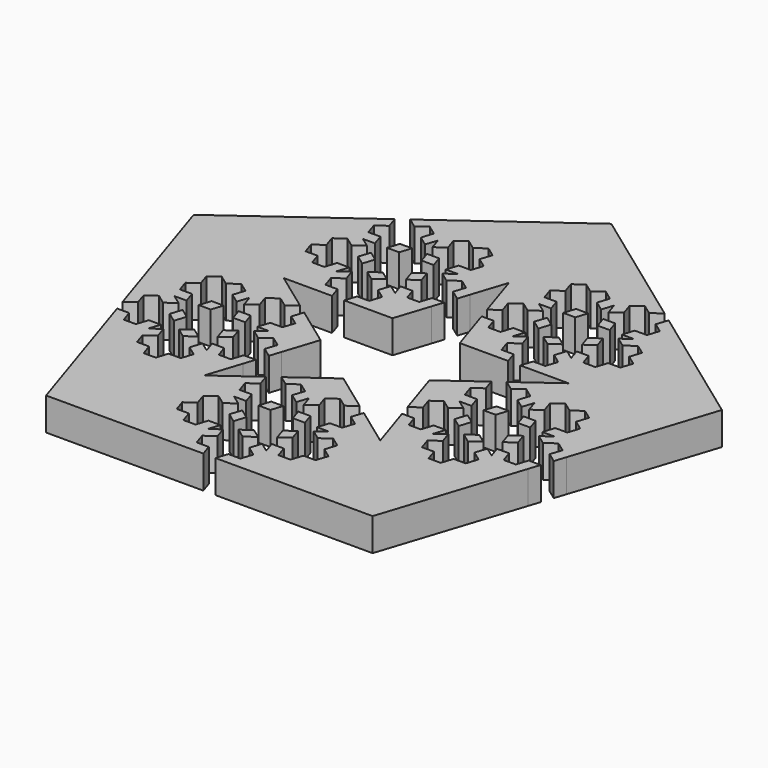
from build123d import *

# Parameters (mm, degrees)
F1_DEPTH = 25.4


with BuildPart() as f1:
    # F0 (on Top) → F1 (new body)
    with BuildSketch(Plane.XY):
        Polygon((45.6645147936, 149.7108812848), (68.4967721904, 166.299487294), (0, 216.0653053214), (-68.4967721904, 166.299487294), (-45.6645147936, 149.7108812848), (-38.053762328, 144.1813459485), (-30.4430098624, 138.6518106121), (-22.8322573968, 133.1222752757), (0, 116.5336692666), (22.8322573968, 133.1222752757), (30.4430098624, 138.6518106121), (38.053762328, 144.1813459485), align=None)
        Polygon((-45.6645147936, 149.7108812848), (-68.4967721904, 166.299487294), (-91.3290295872, 149.7108812848), (-83.7182771216, 144.1813459485), (-76.107524656, 138.6518106121), (-68.4967721904, 133.1222752757), (-60.8860197248, 138.6518106121), (-53.2752672592, 144.1813459485), align=None)
        Polygon((-8.7211462857, 89.6927409178), (0, 116.5336692666), (-22.8322573968, 133.1222752757), (-25.7393061587, 124.1752991594), (-28.6463549206, 115.2283230432), (-31.5534036825, 106.2813469269), (-23.9426512169, 100.7518115905), (-16.3318987513, 95.2222762542), align=None)
        Polygon((25.7393061587, 124.1752991594), (22.8322573968, 133.1222752757), (0, 116.5336692666), (8.7211462857, 89.6927409178), (16.3318987513, 95.2222762542), (23.9426512169, 100.7518115905), (31.5534036825, 106.2813469269), (28.6463549206, 115.2283230432), align=None)
        Polygon((83.7182771216, 144.1813459485), (91.3290295872, 149.7108812848), (68.4967721904, 166.299487294), (45.6645147936, 149.7108812848), (53.2752672592, 144.1813459485), (60.8860197248, 138.6518106121), (68.4967721904, 133.1222752757), (76.107524656, 138.6518106121), align=None)
        Polygon((-83.7182771216, 144.1813459485), (-91.3290295872, 149.7108812848), (-98.9397820528, 144.1813459485), (-91.3290295872, 138.6518106121), align=None)
        Polygon((-68.4967721904, 133.1222752757), (-76.107524656, 138.6518106121), (-79.0145734179, 129.7048344958), (-71.4038209523, 124.1752991594), align=None)
        Polygon((-57.9789709629, 129.7048344958), (-60.8860197248, 138.6518106121), (-68.4967721904, 133.1222752757), (-65.5897234285, 124.1752991594), align=None)
        Polygon((-38.053762328, 144.1813459485), (-45.6645147936, 149.7108812848), (-53.2752672592, 144.1813459485), (-45.6645147936, 138.6518106121), align=None)
        Polygon((-22.8322573968, 133.1222752757), (-30.4430098624, 138.6518106121), (-33.3500586243, 129.7048344958), (-25.7393061587, 124.1752991594), align=None)
        Polygon((-31.5534036825, 106.2813469269), (-28.6463549206, 115.2283230432), (-38.053762328, 115.2283230432), (-40.9608110899, 106.2813469269), align=None)
        Polygon((-31.5534036825, 95.2222762542), (-23.9426512169, 100.7518115905), (-31.5534036825, 106.2813469269), (-39.1641561481, 100.7518115905), align=None)
        Polygon((-11.6281950476, 80.7457648015), (-8.7211462857, 89.6927409178), (-16.3318987513, 95.2222762542), (-19.2389475132, 86.2753001379), align=None)
        Polygon((16.3318987513, 95.2222762542), (8.7211462857, 89.6927409178), (11.6281950476, 80.7457648015), (19.2389475132, 86.2753001379), align=None)
        Polygon((39.1641561481, 100.7518115905), (31.5534036825, 106.2813469269), (23.9426512169, 100.7518115905), (31.5534036825, 95.2222762542), align=None)
        Polygon((38.053762328, 115.2283230432), (28.6463549206, 115.2283230432), (31.5534036825, 106.2813469269), (40.9608110899, 106.2813469269), align=None)
        Polygon((33.3500586243, 129.7048344958), (30.4430098624, 138.6518106121), (22.8322573968, 133.1222752757), (25.7393061587, 124.1752991594), align=None)
        Polygon((53.2752672592, 144.1813459485), (45.6645147936, 149.7108812848), (38.053762328, 144.1813459485), (45.6645147936, 138.6518106121), align=None)
        Polygon((65.5897234285, 124.1752991594), (68.4967721904, 133.1222752757), (60.8860197248, 138.6518106121), (57.9789709629, 129.7048344958), align=None)
        Polygon((79.0145734179, 129.7048344958), (76.107524656, 138.6518106121), (68.4967721904, 133.1222752757), (71.4038209523, 124.1752991594), align=None)
        Polygon((91.3290295872, 138.6518106121), (98.9397820528, 144.1813459485), (91.3290295872, 149.7108812848), (83.7182771216, 144.1813459485), align=None)
    extrude(amount=F1_DEPTH)


with BuildPart() as f1b:
    # F0 (on Top) → F1, piece 2 (new body)
    with BuildSketch(Plane.XY):
        Polygon((156.4946203174, 2.8336722019), (179.3268777142, -13.7549338072), (205.4903165712, 66.7678512391), (136.9935443808, 116.5336692666), (128.2723980951, 89.6927409178), (125.3653493332, 80.7457648015), (122.4583005713, 71.7987886853), (119.5512518094, 62.851812569), (110.8301055237, 36.0108842202), (133.6623629205, 19.4222782111), (141.2731153862, 13.8927428747), (148.8838678518, 8.3632075383), align=None)
        Polygon((128.2723980951, 89.6927409178), (136.9935443808, 116.5336692666), (114.161286984, 133.1222752757), (111.2542382221, 124.1752991594), (108.3471894602, 115.2283230432), (105.4401406983, 106.2813469269), (113.0508931639, 100.7518115905), (120.6616456295, 95.2222762542), align=None)
        Polygon((82.6078833015, 36.0108842202), (110.8301055237, 36.0108842202), (119.5512518094, 62.851812569), (110.143844402, 62.851812569), (100.7364369946, 62.851812569), (91.3290295872, 62.851812569), (88.4219808253, 53.9048364528), (85.5149320634, 44.9578603365), align=None)
        Polygon((126.0516104549, 13.8927428747), (133.6623629205, 19.4222782111), (110.8301055237, 36.0108842202), (87.9978481269, 19.4222782111), (95.6086005925, 13.8927428747), (103.2193530581, 8.3632075383), (110.8301055237, 2.833672202), (118.4408579893, 8.3632075383), align=None)
        Polygon((162.9949789629, -35.0663268196), (170.6057314285, -40.595862156), (179.3268777142, -13.7549338072), (156.4946203174, 2.8336722019), (153.5875715555, -6.1133039143), (150.6805227936, -15.0602800306), (147.7734740317, -24.0072561468), (155.3842264973, -29.5367914832), align=None)
        Polygon((111.2542382221, 124.1752991594), (114.161286984, 133.1222752757), (106.5505345184, 138.6518106121), (103.6434857565, 129.7048344958), align=None)
        Polygon((105.4401406983, 106.2813469269), (108.3471894602, 115.2283230432), (98.9397820528, 115.2283230432), (96.0327332909, 106.2813469269), align=None)
        Polygon((105.4401406983, 95.2222762542), (113.0508931639, 100.7518115905), (105.4401406983, 106.2813469269), (97.8293882327, 100.7518115905), align=None)
        Polygon((125.3653493332, 80.7457648015), (128.2723980951, 89.6927409178), (120.6616456295, 95.2222762542), (117.7545968676, 86.2753001379), align=None)
        Polygon((119.5512518094, 62.851812569), (122.4583005713, 71.7987886853), (113.0508931639, 71.7987886853), (110.143844402, 62.851812569), align=None)
        Polygon((91.3290295872, 62.851812569), (100.7364369946, 62.851812569), (97.8293882327, 71.7987886853), (88.4219808253, 71.7987886853), align=None)
        Polygon((80.8112283597, 59.4343717891), (88.4219808253, 53.9048364528), (91.3290295872, 62.851812569), (83.7182771216, 68.3813479054), align=None)
        Polygon((73.2004758941, 36.0108842202), (82.6078833015, 36.0108842202), (85.5149320634, 44.9578603365), (76.107524656, 44.9578603365), align=None)
        Polygon((95.6086005925, 13.8927428747), (87.9978481269, 19.4222782111), (80.3870956613, 13.8927428747), (87.9978481269, 8.3632075383), align=None)
        Polygon((107.9230567618, -6.1133039143), (110.8301055237, 2.833672202), (103.2193530581, 8.3632075383), (100.3123042962, -0.5837685779), align=None)
        Polygon((121.3479067512, -0.5837685779), (118.4408579893, 8.3632075383), (110.8301055237, 2.833672202), (113.7371542856, -6.1133039143), align=None)
        Polygon((133.6623629205, 8.3632075383), (141.2731153862, 13.8927428747), (133.6623629205, 19.4222782111), (126.0516104549, 13.8927428747), align=None)
        Polygon((153.5875715555, -6.1133039143), (156.4946203174, 2.833672202), (148.8838678518, 8.3632075383), (145.9768190899, -0.5837685779), align=None)
        Polygon((138.3660666243, -24.0072561468), (147.7734740317, -24.0072561468), (150.6805227936, -15.0602800306), (141.2731153862, -15.0602800306), align=None)
        Polygon((147.7734740317, -35.0663268196), (155.3842264973, -29.5367914832), (147.7734740317, -24.0072561468), (140.1627215661, -29.5367914832), align=None)
        Polygon((160.087930201, -44.0133029358), (167.6986826666, -49.5428382722), (170.6057314285, -40.595862156), (162.9949789629, -35.0663268196), align=None)
    extrude(amount=F1_DEPTH)


with BuildPart() as f1c:
    # F0 (on Top) → F1, piece 3 (new body)
    with BuildSketch(Plane.XY):
        Polygon((42.3333333333, -174.8005038998), (127, -174.8005038998), (153.1634388571, -94.2777188535), (124.9412166349, -94.2777188535), (115.5338092274, -94.2777188535), (106.12640182, -94.2777188535), (96.7189944126, -94.2777188535), (68.4967721904, -94.2777188535), (59.7756259047, -121.1186472023), (56.8685771428, -130.0656233185), (53.9615283809, -139.0125994348), (51.054479619, -147.9595755511), align=None)
        Polygon((124.9412166349, -94.2777188535), (153.1634388571, -94.2777188535), (161.8845851428, -67.4367905047), (152.4771777354, -67.4367905047), (143.069770328, -67.4367905047), (133.6623629205, -67.4367905047), (130.7553141587, -76.383766621), (127.8482653968, -85.3307427373), align=None)
        Polygon((68.4967721904, -94.2777188535), (96.7189944126, -94.2777188535), (93.8119456507, -85.3307427373), (90.9048968888, -76.383766621), (87.9978481269, -67.4367905047), (78.5904407195, -67.4367905047), (69.1830333121, -67.4367905047), (59.7756259047, -67.4367905047), align=None)
        Polygon((52.1648734391, -115.5891118659), (59.7756259047, -121.1186472023), (68.4967721904, -94.2777188535), (45.6645147936, -77.6891128444), (42.7574660317, -86.6360889606), (39.8504172698, -95.5830650769), (36.9433685079, -104.5300411931), (44.5541209735, -110.0595765295), align=None)
        Polygon((14.1111111111, -174.8005038998), (42.3333333333, -174.8005038998), (51.054479619, -147.9595755511), (41.6470722116, -147.9595755511), (32.2396648042, -147.9595755511), (22.8322573968, -147.9595755511), (19.9252086349, -156.9065516673), (17.018159873, -165.8535277836), align=None)
        Polygon((152.4771777354, -67.4367905047), (161.8845851428, -67.4367905047), (164.7916339047, -58.4898143885), (155.3842264973, -58.4898143885), align=None)
        Polygon((133.6623629205, -67.4367905047), (143.069770328, -67.4367905047), (140.1627215661, -58.4898143885), (130.7553141587, -58.4898143885), align=None)
        Polygon((123.1445616931, -70.8542312846), (130.7553141587, -76.383766621), (133.6623629205, -67.4367905047), (126.0516104549, -61.9072551684), align=None)
        Polygon((115.5338092274, -94.2777188535), (124.9412166349, -94.2777188535), (127.8482653968, -85.3307427373), (118.4408579893, -85.3307427373), align=None)
        Polygon((96.7189944126, -94.2777188535), (106.12640182, -94.2777188535), (103.2193530581, -85.3307427373), (93.8119456507, -85.3307427373), align=None)
        Polygon((87.9978481269, -67.4367905047), (90.9048968888, -76.383766621), (98.5156493544, -70.8542312846), (95.6086005925, -61.9072551684), align=None)
        Polygon((78.5904407195, -67.4367905047), (87.9978481269, -67.4367905047), (90.9048968888, -58.4898143885), (81.4974894814, -58.4898143885), align=None)
        Polygon((56.8685771428, -58.4898143885), (59.7756259047, -67.4367905047), (69.1830333121, -67.4367905047), (66.2759845502, -58.4898143885), align=None)
        Polygon((42.7574660317, -86.6360889606), (45.6645147936, -77.6891128444), (38.053762328, -72.159577508), (35.1467135661, -81.1065536242), align=None)
        Polygon((27.5359611005, -104.5300411931), (36.9433685079, -104.5300411931), (39.8504172698, -95.5830650769), (30.4430098624, -95.5830650769), align=None)
        Polygon((36.9433685079, -115.5891118659), (44.5541209735, -110.0595765295), (36.9433685079, -104.5300411931), (29.3326160423, -110.0595765295), align=None)
        Polygon((49.2578246772, -124.5360879822), (56.8685771428, -130.0656233185), (59.7756259047, -121.1186472023), (52.1648734391, -115.5891118659), align=None)
        Polygon((41.6470722116, -147.9595755511), (51.054479619, -147.9595755511), (53.9615283809, -139.0125994348), (44.5541209735, -139.0125994348), align=None)
        Polygon((22.8322573968, -147.9595755511), (32.2396648042, -147.9595755511), (29.3326160423, -139.0125994348), (19.9252086349, -139.0125994348), align=None)
        Polygon((12.3144561693, -151.3770163309), (19.9252086349, -156.9065516673), (22.8322573968, -147.9595755511), (15.2215049312, -142.4300402147), align=None)
        Polygon((4.7037037037, -174.8005038998), (14.1111111111, -174.8005038998), (17.018159873, -165.8535277836), (7.6107524656, -165.8535277836), align=None)
    extrude(amount=F1_DEPTH)


with BuildPart() as f1d:
    # F0 (on Top) → F1, piece 4 (new body)
    with BuildSketch(Plane.XY):
        Polygon((-127, -174.8005038998), (-42.3333333333, -174.8005038998), (-51.054479619, -147.9595755511), (-53.9615283809, -139.0125994348), (-56.8685771428, -130.0656233185), (-59.7756259047, -121.1186472023), (-68.4967721904, -94.2777188535), (-96.7189944126, -94.2777188535), (-106.12640182, -94.2777188535), (-115.5338092274, -94.2777188535), (-124.9412166349, -94.2777188535), (-153.1634388571, -94.2777188535), align=None)
        Polygon((-42.3333333333, -174.8005038998), (-14.1111111111, -174.8005038998), (-17.018159873, -165.8535277836), (-19.9252086349, -156.9065516673), (-22.8322573968, -147.9595755511), (-32.2396648042, -147.9595755511), (-41.6470722116, -147.9595755511), (-51.054479619, -147.9595755511), align=None)
        Polygon((-68.4967721904, -94.2777188535), (-59.7756259047, -121.1186472023), (-52.1648734391, -115.5891118659), (-44.5541209735, -110.0595765295), (-36.9433685079, -104.5300411931), (-39.8504172698, -95.5830650769), (-42.7574660317, -86.6360889606), (-45.6645147936, -77.6891128444), align=None)
        Polygon((-96.7189944126, -94.2777188535), (-68.4967721904, -94.2777188535), (-59.7756259047, -67.4367905047), (-69.1830333121, -67.4367905047), (-78.5904407195, -67.4367905047), (-87.9978481269, -67.4367905047), (-90.9048968888, -76.383766621), (-93.8119456507, -85.3307427373), align=None)
        Polygon((-161.8845851428, -67.4367905047), (-153.1634388571, -94.2777188535), (-124.9412166349, -94.2777188535), (-127.8482653968, -85.3307427373), (-130.7553141587, -76.383766621), (-133.6623629205, -67.4367905047), (-143.069770328, -67.4367905047), (-152.4771777354, -67.4367905047), align=None)
        Polygon((-14.1111111111, -174.8005038998), (-4.7037037037, -174.8005038998), (-7.6107524656, -165.8535277836), (-17.018159873, -165.8535277836), align=None)
        Polygon((-22.8322573968, -147.9595755511), (-19.9252086349, -156.9065516673), (-12.3144561693, -151.3770163309), (-15.2215049312, -142.4300402147), align=None)
        Polygon((-32.2396648042, -147.9595755511), (-22.8322573968, -147.9595755511), (-19.9252086349, -139.0125994348), (-29.3326160423, -139.0125994348), align=None)
        Polygon((-53.9615283809, -139.0125994348), (-51.054479619, -147.9595755511), (-41.6470722116, -147.9595755511), (-44.5541209735, -139.0125994348), align=None)
        Polygon((-59.7756259047, -121.1186472023), (-56.8685771428, -130.0656233185), (-49.2578246772, -124.5360879822), (-52.1648734391, -115.5891118659), align=None)
        Polygon((-36.9433685079, -104.5300411931), (-44.5541209735, -110.0595765295), (-36.9433685079, -115.5891118659), (-29.3326160423, -110.0595765295), align=None)
        Polygon((-39.8504172698, -95.5830650769), (-36.9433685079, -104.5300411931), (-27.5359611005, -104.5300411931), (-30.4430098624, -95.5830650769), align=None)
        Polygon((-38.053762328, -72.159577508), (-45.6645147936, -77.6891128444), (-42.7574660317, -86.6360889606), (-35.1467135661, -81.1065536243), align=None)
        Polygon((-140.1627215661, -58.4898143885), (-143.069770328, -67.4367905047), (-133.6623629205, -67.4367905047), (-130.7553141587, -58.4898143885), align=None)
        Polygon((-164.7916339047, -58.4898143885), (-161.8845851428, -67.4367905047), (-152.4771777354, -67.4367905047), (-155.3842264973, -58.4898143885), align=None)
        Polygon((-87.9978481269, -67.4367905047), (-78.5904407195, -67.4367905047), (-81.4974894814, -58.4898143885), (-90.9048968888, -58.4898143885), align=None)
        Polygon((-69.1830333121, -67.4367905047), (-59.7756259047, -67.4367905047), (-56.8685771428, -58.4898143885), (-66.2759845502, -58.4898143885), align=None)
        Polygon((-103.2193530581, -85.3307427373), (-106.12640182, -94.2777188535), (-96.7189944126, -94.2777188535), (-93.8119456507, -85.3307427373), align=None)
        Polygon((-127.8482653968, -85.3307427373), (-124.9412166349, -94.2777188535), (-115.5338092274, -94.2777188535), (-118.4408579893, -85.3307427373), align=None)
        Polygon((-133.6623629205, -67.4367905047), (-130.7553141587, -76.383766621), (-123.1445616931, -70.8542312846), (-126.0516104549, -61.9072551684), align=None)
        Polygon((-98.5156493544, -70.8542312846), (-90.9048968888, -76.383766621), (-87.9978481269, -67.4367905047), (-95.6086005925, -61.9072551684), align=None)
    extrude(amount=F1_DEPTH)


with BuildPart() as f1e:
    # F0 (on Top) → F1, piece 5 (new body)
    with BuildSketch(Plane.XY):
        Polygon((-205.4903165712, 66.7678512391), (-179.3268777142, -13.7549338072), (-156.4946203174, 2.833672202), (-148.8838678518, 8.3632075383), (-141.2731153862, 13.8927428747), (-133.6623629205, 19.4222782111), (-110.8301055237, 36.0108842202), (-119.5512518094, 62.851812569), (-122.4583005713, 71.7987886853), (-125.3653493332, 80.7457648015), (-128.2723980951, 89.6927409178), (-136.9935443808, 116.5336692666), align=None)
        Polygon((-114.161286984, 133.1222752757), (-136.9935443808, 116.5336692666), (-128.2723980951, 89.6927409178), (-120.6616456295, 95.2222762542), (-113.0508931639, 100.7518115905), (-105.4401406983, 106.2813469269), (-108.3471894602, 115.2283230432), (-111.2542382221, 124.1752991594), align=None)
        Polygon((-179.3268777142, -13.7549338072), (-170.6057314285, -40.595862156), (-162.9949789629, -35.0663268196), (-155.3842264973, -29.5367914832), (-147.7734740317, -24.0072561468), (-150.6805227936, -15.0602800306), (-153.5875715555, -6.1133039143), (-156.4946203174, 2.833672202), align=None)
        Polygon((-110.8301055237, 36.0108842202), (-133.6623629205, 19.4222782111), (-126.0516104549, 13.8927428747), (-118.4408579893, 8.3632075383), (-110.8301055237, 2.833672202), (-103.2193530581, 8.3632075383), (-95.6086005925, 13.8927428747), (-87.9978481269, 19.4222782111), align=None)
        Polygon((-119.5512518094, 62.851812569), (-110.8301055237, 36.0108842202), (-82.6078833015, 36.0108842202), (-85.5149320634, 44.9578603365), (-88.4219808253, 53.9048364528), (-91.3290295872, 62.851812569), (-100.7364369946, 62.851812569), (-110.143844402, 62.851812569), align=None)
        Polygon((-106.5505345184, 138.6518106121), (-114.161286984, 133.1222752757), (-111.2542382221, 124.1752991594), (-103.6434857565, 129.7048344958), align=None)
        Polygon((-98.9397820528, 115.2283230432), (-108.3471894602, 115.2283230432), (-105.4401406983, 106.2813469269), (-96.0327332909, 106.2813469269), align=None)
        Polygon((-105.4401406983, 106.2813469269), (-113.0508931639, 100.7518115905), (-105.4401406983, 95.2222762542), (-97.8293882327, 100.7518115905), align=None)
        Polygon((-120.6616456295, 95.2222762542), (-128.2723980951, 89.6927409178), (-125.3653493332, 80.7457648015), (-117.7545968676, 86.2753001379), align=None)
        Polygon((-113.0508931639, 71.7987886853), (-122.4583005713, 71.7987886853), (-119.5512518094, 62.851812569), (-110.143844402, 62.851812569), align=None)
        Polygon((-97.8293882327, 71.7987886853), (-100.7364369946, 62.851812569), (-91.3290295872, 62.851812569), (-88.4219808253, 71.7987886853), align=None)
        Polygon((-91.3290295872, 62.851812569), (-88.4219808253, 53.9048364528), (-80.8112283597, 59.4343717891), (-83.7182771216, 68.3813479054), align=None)
        Polygon((-85.5149320634, 44.9578603365), (-82.6078833015, 36.0108842202), (-73.2004758941, 36.0108842202), (-76.107524656, 44.9578603365), align=None)
        Polygon((-170.6057314285, -40.595862156), (-167.6986826666, -49.5428382722), (-160.087930201, -44.0133029358), (-162.9949789629, -35.0663268196), align=None)
        Polygon((-147.7734740317, -24.0072561468), (-155.3842264973, -29.5367914832), (-147.7734740317, -35.0663268196), (-140.1627215661, -29.5367914832), align=None)
        Polygon((-150.6805227936, -15.0602800306), (-147.7734740317, -24.0072561468), (-138.3660666243, -24.0072561468), (-141.2731153862, -15.0602800306), align=None)
        Polygon((-148.8838678518, 8.3632075383), (-156.4946203174, 2.833672202), (-153.5875715555, -6.1133039143), (-145.9768190899, -0.5837685779), align=None)
        Polygon((-133.6623629205, 19.4222782111), (-141.2731153862, 13.8927428747), (-133.6623629205, 8.3632075383), (-126.0516104549, 13.8927428747), align=None)
        Polygon((-110.8301055237, 2.833672202), (-118.4408579893, 8.3632075383), (-121.3479067512, -0.5837685779), (-113.7371542856, -6.1133039143), align=None)
        Polygon((-103.2193530581, 8.3632075383), (-110.8301055237, 2.833672202), (-107.9230567618, -6.1133039143), (-100.3123042962, -0.5837685779), align=None)
        Polygon((-80.3870956613, 13.8927428747), (-87.9978481269, 19.4222782111), (-95.6086005925, 13.8927428747), (-87.9978481269, 8.3632075383), align=None)
    extrude(amount=F1_DEPTH)


with BuildPart() as f1f:
    # F0 (on Top) → F1, piece 6 (new body)
    with BuildSketch(Plane.XY):
        Polygon((-51.4786123174, 44.9578603365), (-54.3856610793, 36.0108842202), (-26.1634388571, 36.0108842202), (-17.4422925714, 62.851812569), (-26.8496999788, 62.851812569), (-36.2571073862, 62.851812569), (-45.6645147936, 62.851812569), (-48.5715635555, 53.9048364528), align=None)
        Polygon((-17.4422925714, 62.851812569), (-14.5352438095, 71.7987886853), (-23.9426512169, 71.7987886853), (-26.8496999788, 62.851812569), align=None)
        Polygon((-45.6645147936, 62.851812569), (-36.2571073862, 62.851812569), (-39.1641561481, 71.7987886853), (-48.5715635555, 71.7987886853), align=None)
        Polygon((-56.1823160211, 59.4343717891), (-48.5715635555, 53.9048364528), (-45.6645147936, 62.851812569), (-53.2752672592, 68.3813479054), align=None)
        Polygon((-60.8860197248, 44.9578603365), (-63.7930684867, 36.0108842202), (-54.3856610793, 36.0108842202), (-51.4786123174, 44.9578603365), align=None)
    extrude(amount=F1_DEPTH)


with BuildPart() as f1g:
    # F0 (on Top) → F1, piece 7 (new body)
    with BuildSketch(Plane.XY):
        Polygon((26.1634388571, 36.0108842202), (54.3856610793, 36.0108842202), (51.4786123174, 44.9578603365), (48.5715635555, 53.9048364528), (45.6645147936, 62.851812569), (36.2571073862, 62.851812569), (26.8496999788, 62.851812569), (17.4422925714, 62.851812569), align=None)
        Polygon((54.3856610793, 36.0108842202), (63.7930684867, 36.0108842202), (60.8860197248, 44.9578603365), (51.4786123174, 44.9578603365), align=None)
        Polygon((45.6645147936, 62.851812569), (48.5715635555, 53.9048364528), (56.1823160211, 59.4343717891), (53.2752672592, 68.3813479054), align=None)
        Polygon((36.2571073862, 62.851812569), (45.6645147936, 62.851812569), (48.5715635555, 71.7987886853), (39.1641561481, 71.7987886853), align=None)
        Polygon((14.5352438095, 71.7987886853), (17.4422925714, 62.851812569), (26.8496999788, 62.851812569), (23.9426512169, 71.7987886853), align=None)
    extrude(amount=F1_DEPTH)


with BuildPart() as f1h:
    # F0 (on Top) → F1, piece 8 (new body)
    with BuildSketch(Plane.XY):
        Polygon((42.3333333333, -13.7549338072), (51.054479619, -40.595862156), (58.6652320846, -35.0663268196), (66.2759845502, -29.5367914832), (73.8867370158, -24.0072561468), (70.9796882539, -15.0602800306), (68.072639492, -6.1133039143), (65.1655907301, 2.833672202), align=None)
        Polygon((51.054479619, -40.595862156), (53.9615283809, -49.5428382722), (61.5722808465, -44.0133029358), (58.6652320846, -35.0663268196), align=None)
        Polygon((73.8867370158, -24.0072561468), (66.2759845502, -29.5367914832), (73.8867370158, -35.0663268196), (81.4974894814, -29.5367914832), align=None)
        Polygon((70.9796882539, -15.0602800306), (73.8867370158, -24.0072561468), (83.2941444232, -24.0072561468), (80.3870956613, -15.0602800306), align=None)
        Polygon((72.7763431957, 8.3632075383), (65.1655907301, 2.833672202), (68.072639492, -6.1133039143), (75.6833919576, -0.5837685779), align=None)
    extrude(amount=F1_DEPTH)


with BuildPart() as f1i:
    # F0 (on Top) → F1, piece 9 (new body)
    with BuildSketch(Plane.XY):
        Polygon((15.2215049312, -66.6300421716), (22.8322573968, -61.1005068352), (0, -44.5119008261), (-22.8322573968, -61.1005068352), (-15.2215049312, -66.6300421716), (-7.6107524656, -72.159577508), (0, -77.6891128444), (7.6107524656, -72.159577508), align=None)
        Polygon((22.8322573968, -72.159577508), (30.4430098624, -66.6300421716), (22.8322573968, -61.1005068352), (15.2215049312, -66.6300421716), align=None)
        Polygon((-15.2215049312, -66.6300421716), (-22.8322573968, -61.1005068352), (-30.4430098624, -66.6300421716), (-22.8322573968, -72.159577508), align=None)
        Polygon((-2.9070487619, -86.6360889606), (0, -77.6891128444), (-7.6107524656, -72.159577508), (-10.5178012275, -81.1065536242), align=None)
        Polygon((10.5178012275, -81.1065536242), (7.6107524656, -72.159577508), (0, -77.6891128444), (2.9070487619, -86.6360889606), align=None)
    extrude(amount=F1_DEPTH)


with BuildPart() as f1j:
    # F0 (on Top) → F1, piece 10 (new body)
    with BuildSketch(Plane.XY):
        Polygon((-58.6652320846, -35.0663268196), (-51.054479619, -40.595862156), (-42.3333333333, -13.7549338072), (-65.1655907301, 2.833672202), (-68.072639492, -6.1133039143), (-70.9796882539, -15.0602800306), (-73.8867370158, -24.0072561468), (-66.2759845502, -29.5367914832), align=None)
        Polygon((-68.072639492, -6.1133039143), (-65.1655907301, 2.833672202), (-72.7763431957, 8.3632075383), (-75.6833919576, -0.5837685779), align=None)
        Polygon((-83.2941444232, -24.0072561468), (-73.8867370158, -24.0072561468), (-70.9796882539, -15.0602800306), (-80.3870956613, -15.0602800306), align=None)
        Polygon((-73.8867370158, -35.0663268196), (-66.2759845502, -29.5367914832), (-73.8867370158, -24.0072561468), (-81.4974894814, -29.5367914832), align=None)
        Polygon((-61.5722808465, -44.0133029358), (-53.9615283809, -49.5428382722), (-51.054479619, -40.595862156), (-58.6652320846, -35.0663268196), align=None)
    extrude(amount=F1_DEPTH)


with BuildPart() as f1k:
    # F0 (on Top) → F1, piece 11 (new body)
    with BuildSketch(Plane.XY):
        Polygon((59.7756259047, 106.2813469269), (62.6826746666, 115.2283230432), (53.2752672592, 115.2283230432), (50.3682184973, 106.2813469269), align=None)
    extrude(amount=F1_DEPTH)


with BuildPart() as f1l:
    # F0 (on Top) → F1, piece 12 (new body)
    with BuildSketch(Plane.XY):
        Polygon((86.6253258835, 106.2813469269), (83.7182771216, 115.2283230432), (74.3108697142, 115.2283230432), (77.2179184761, 106.2813469269), align=None)
    extrude(amount=F1_DEPTH)


with BuildPart() as f1m:
    # F0 (on Top) → F1, piece 13 (new body)
    with BuildSketch(Plane.XY):
        Polygon((93.125684529, 86.2753001379), (90.2186357671, 95.2222762542), (82.6078833015, 89.6927409178), (85.5149320634, 80.7457648015), align=None)
    extrude(amount=F1_DEPTH)


with BuildPart() as f1n:
    # F0 (on Top) → F1, piece 14 (new body)
    with BuildSketch(Plane.XY):
        Polygon((68.4967721904, 68.3813479054), (76.107524656, 73.9108832418), (68.4967721904, 79.4404185782), (60.8860197248, 73.9108832418), align=None)
    extrude(amount=F1_DEPTH)


with BuildPart() as f1o:
    # F0 (on Top) → F1, piece 15 (new body)
    with BuildSketch(Plane.XY):
        Polygon((43.8678598518, 86.2753001379), (51.4786123174, 80.7457648015), (54.3856610793, 89.6927409178), (46.7749086137, 95.2222762542), align=None)
    extrude(amount=F1_DEPTH)


with BuildPart() as f1p:
    # F0 (on Top) → F1, piece 16 (new body)
    with BuildSketch(Plane.XY):
        Polygon((-43.8678598518, 86.2753001379), (-46.7749086137, 95.2222762542), (-54.3856610793, 89.6927409178), (-51.4786123174, 80.7457648015), align=None)
    extrude(amount=F1_DEPTH)


with BuildPart() as f1q:
    # F0 (on Top) → F1, piece 17 (new body)
    with BuildSketch(Plane.XY):
        Polygon((-53.2752672592, 115.2283230432), (-62.6826746666, 115.2283230432), (-59.7756259047, 106.2813469269), (-50.3682184973, 106.2813469269), align=None)
    extrude(amount=F1_DEPTH)


with BuildPart() as f1r:
    # F0 (on Top) → F1, piece 18 (new body)
    with BuildSketch(Plane.XY):
        Polygon((-74.3108697142, 115.2283230432), (-83.7182771216, 115.2283230432), (-86.6253258835, 106.2813469269), (-77.2179184761, 106.2813469269), align=None)
    extrude(amount=F1_DEPTH)


with BuildPart() as f1s:
    # F0 (on Top) → F1, piece 19 (new body)
    with BuildSketch(Plane.XY):
        Polygon((-82.6078833015, 89.6927409178), (-90.2186357671, 95.2222762542), (-93.125684529, 86.2753001379), (-85.5149320634, 80.7457648015), align=None)
    extrude(amount=F1_DEPTH)


with BuildPart() as f1t:
    # F0 (on Top) → F1, piece 20 (new body)
    with BuildSketch(Plane.XY):
        Polygon((-68.4967721904, 79.4404185782), (-76.107524656, 73.9108832418), (-68.4967721904, 68.3813479054), (-60.8860197248, 73.9108832418), align=None)
    extrude(amount=F1_DEPTH)


with BuildPart() as f1u:
    # F0 (on Top) → F1, piece 21 (new body)
    with BuildSketch(Plane.XY):
        Polygon((95.6086005925, -15.0602800306), (92.7015518306, -24.0072561468), (102.1089592381, -24.0072561468), (105.016008, -15.0602800306), align=None)
    extrude(amount=F1_DEPTH)


with BuildPart() as f1v:
    # F0 (on Top) → F1, piece 22 (new body)
    with BuildSketch(Plane.XY):
        Polygon((119.5512518094, -24.0072561468), (128.9586592168, -24.0072561468), (126.0516104549, -15.0602800306), (116.6442030475, -15.0602800306), align=None)
    extrude(amount=F1_DEPTH)


with BuildPart() as f1w:
    # F0 (on Top) → F1, piece 23 (new body)
    with BuildSketch(Plane.XY):
        Polygon((127.8482653968, -49.5428382722), (135.4590178624, -44.0133029358), (132.5519691005, -35.0663268196), (124.9412166349, -40.595862156), align=None)
    extrude(amount=F1_DEPTH)


with BuildPart() as f1x:
    # F0 (on Top) → F1, piece 24 (new body)
    with BuildSketch(Plane.XY):
        Polygon((110.8301055237, -61.9072551684), (118.4408579893, -56.377719832), (110.8301055237, -50.8481844956), (103.2193530581, -56.377719832), align=None)
    extrude(amount=F1_DEPTH)


with BuildPart() as f1y:
    # F0 (on Top) → F1, piece 25 (new body)
    with BuildSketch(Plane.XY):
        Polygon((86.2011931851, -44.0133029358), (93.8119456507, -49.5428382722), (96.7189944126, -40.595862156), (89.108241947, -35.0663268196), align=None)
    extrude(amount=F1_DEPTH)


with BuildPart() as f1z:
    # F0 (on Top) → F1, piece 26 (new body)
    with BuildSketch(Plane.XY):
        Polygon((14.1111111111, -121.1186472023), (17.018159873, -130.0656233185), (24.6289123386, -124.5360879822), (21.7218635767, -115.5891118659), align=None)
    extrude(amount=F1_DEPTH)


with BuildPart() as f1ba:
    # F0 (on Top) → F1, piece 27 (new body)
    with BuildSketch(Plane.XY):
        Polygon((0, -142.4300402147), (7.6107524656, -136.9005048783), (0, -131.3709695419), (-7.6107524656, -136.9005048783), align=None)
    extrude(amount=F1_DEPTH)


with BuildPart() as f1bb:
    # F0 (on Top) → F1, piece 28 (new body)
    with BuildSketch(Plane.XY):
        Polygon((-24.6289123386, -124.5360879822), (-17.018159873, -130.0656233185), (-14.1111111111, -121.1186472023), (-21.7218635767, -115.5891118659), align=None)
    extrude(amount=F1_DEPTH)


with BuildPart() as f1bc:
    # F0 (on Top) → F1, piece 29 (new body)
    with BuildSketch(Plane.XY):
        Polygon((-15.2215049312, -95.5830650769), (-18.1285536931, -104.5300411931), (-8.7211462857, -104.5300411931), (-5.8140975238, -95.5830650769), align=None)
    extrude(amount=F1_DEPTH)


with BuildPart() as f1bd:
    # F0 (on Top) → F1, piece 30 (new body)
    with BuildSketch(Plane.XY):
        Polygon((8.7211462857, -104.5300411931), (18.1285536931, -104.5300411931), (15.2215049312, -95.5830650769), (5.8140975238, -95.5830650769), align=None)
    extrude(amount=F1_DEPTH)


with BuildPart() as f1be:
    # F0 (on Top) → F1, piece 31 (new body)
    with BuildSketch(Plane.XY):
        Polygon((-132.5519691005, -35.0663268196), (-135.4590178624, -44.0133029358), (-127.8482653968, -49.5428382722), (-124.9412166349, -40.595862156), align=None)
    extrude(amount=F1_DEPTH)


with BuildPart() as f1bf:
    # F0 (on Top) → F1, piece 32 (new body)
    with BuildSketch(Plane.XY):
        Polygon((-126.0516104549, -15.0602800306), (-128.9586592168, -24.0072561468), (-119.5512518094, -24.0072561468), (-116.6442030475, -15.0602800306), align=None)
    extrude(amount=F1_DEPTH)


with BuildPart() as f1bg:
    # F0 (on Top) → F1, piece 33 (new body)
    with BuildSketch(Plane.XY):
        Polygon((-102.1089592381, -24.0072561468), (-92.7015518306, -24.0072561468), (-95.6086005925, -15.0602800306), (-105.016008, -15.0602800306), align=None)
    extrude(amount=F1_DEPTH)


with BuildPart() as f1bh:
    # F0 (on Top) → F1, piece 34 (new body)
    with BuildSketch(Plane.XY):
        Polygon((-96.7189944126, -40.595862156), (-93.8119456507, -49.5428382722), (-86.2011931851, -44.0133029358), (-89.108241947, -35.0663268196), align=None)
    extrude(amount=F1_DEPTH)


with BuildPart() as f1bi:
    # F0 (on Top) → F1, piece 35 (new body)
    with BuildSketch(Plane.XY):
        Polygon((-110.8301055237, -50.8481844956), (-118.4408579893, -56.377719832), (-110.8301055237, -61.9072551684), (-103.2193530581, -56.377719832), align=None)
    extrude(amount=F1_DEPTH)


solid = Compound([f1.part, f1b.part, f1c.part, f1d.part, f1e.part, f1f.part, f1g.part, f1h.part, f1i.part, f1j.part, f1k.part, f1l.part, f1m.part, f1n.part, f1o.part, f1p.part, f1q.part, f1r.part, f1s.part, f1t.part, f1u.part, f1v.part, f1w.part, f1x.part, f1y.part, f1z.part, f1ba.part, f1bb.part, f1bc.part, f1bd.part, f1be.part, f1bf.part, f1bg.part, f1bh.part, f1bi.part])
